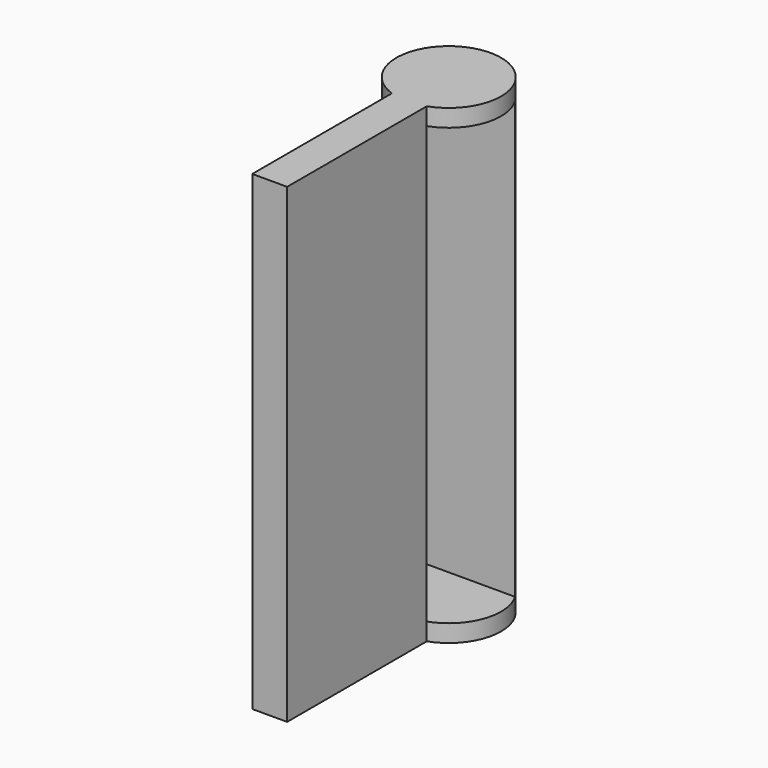
from build123d import *

# Parameters (mm, degrees)
F1_DEPTH = 27
F2_W     = 4.3404353922
F2_H     = 25
F3_DEPTH = 25


# Not quite as in the source:
# - a feature names something its author has since deleted; it is built from what else it names


with BuildPart() as f1:
    # F0 (on Top) → F1 (new body)
    with BuildSketch(Plane.XY):
        with BuildLine():
            Line((-9.8292995244, 17.7390783057), (-9.8292995244, 7.7390783057))
            Line((-9.8292995244, 7.7390783057), (-7.8292995244, 7.7390783057))
            Line((-7.8292995244, 7.7390783057), (-7.8292995244, 17.7390783057))
            ThreePointArc((-7.8292995244, 17.7390783057), (-8.8292995244, 23.5675054304), (-9.8292995244, 17.7390783057))
        make_face()
    extrude(amount=F1_DEPTH)

    # F2 (on Right) → F3 (cut)
    with BuildSketch(Plane.YZ):
        with Locations((19.9092960018, 13.5)):
            Rectangle(F2_W, F2_H)
    extrude(amount=-F3_DEPTH, mode=Mode.SUBTRACT)


solid = f1.part
